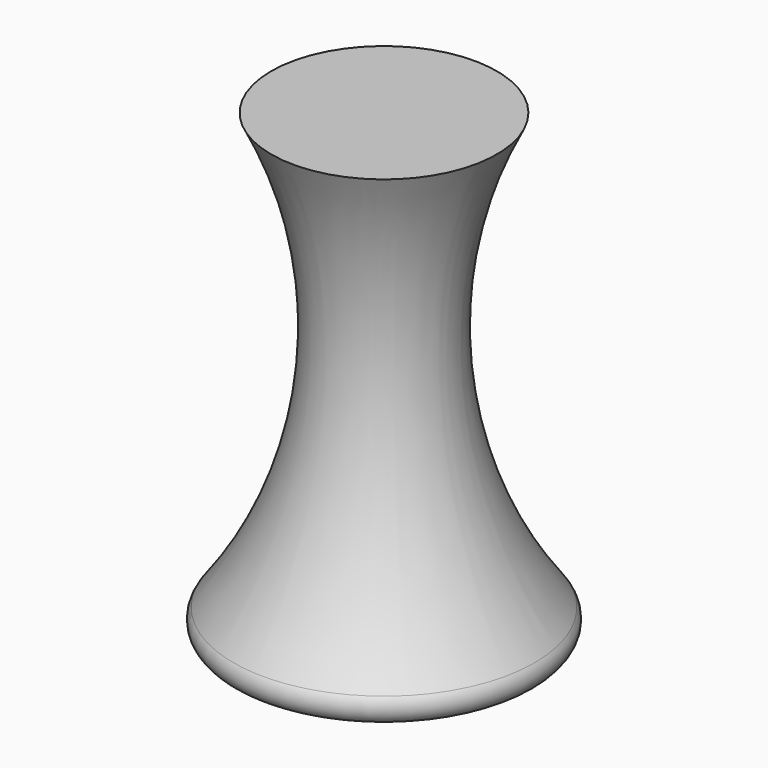
from build123d import *

# Parameters (mm, degrees)
F2_T = -7.62
F4_R = 5.08


# Not quite as in the source:
# - a fillet or chamfer that OpenCascade refuses, or shapes differently, is made with other operations: its cross-section is extruded or revolved along the edge and cut away or added


with BuildPart() as f1:
    # F0 (on Front) → F1 (revolve)
    with BuildSketch(Plane.XZ):
        with BuildLine():
            Line((143.8946140909, -50.2851232886), (143.8946140909, 51.3148767114))
            Line((143.8946140909, 51.3148767114), (119.1407005906, 51.3148767114))
            ThreePointArc((119.1407005906, 51.3148767114), (128.4046098857, -1.5785873359), (105.7946140909, -50.2851232886))
            Line((105.7946140909, -50.2851232886), (143.8946140909, -50.2851232886))
        make_face()
    revolve(axis=Axis((143.8946140909, 0, 0.5148767114), (0, 0, -1)))

    # F2
    f2_openings = [f1.faces().sort_by_distance(p)[0] for p in [
        (143.894614, 0, -50.285123),
    ]]
    offset(amount=F2_T, openings=f2_openings)

    # F3: fillet of radius 3.81 on 2 edges, made by hand

    # F3_s1 → F3_t2 (revolve, cut)
    with BuildSketch(Plane.XZ):
        with BuildLine():
            ThreePointArc((113.9178982469, -50.2855232886), (115.6120189188, -49.8884342421), (116.9532297374, -48.7798864977))
            Line((116.9532297374, -48.7798864977), (117.2567628865, -49.0105628186))
            ThreePointArc((117.2567628865, -49.0105628186), (116.6740859752, -49.7688758954), (116.0843279253, -50.5216973629))
            Line((116.0843279253, -50.5216973629), (115.7853686555, -50.6663632886))
            ThreePointArc((115.7853686555, -50.6663632886), (114.8516334512, -50.6663632886), (113.9178982469, -50.6667632886))
            Line((113.9178982469, -50.6667632886), (113.9178982469, -50.2855232886))
        make_face()
    revolve(axis=Axis((143.8946140909, 0, -50.2851232886), (0, 0, 1)), mode=Mode.SUBTRACT)

    # F3_s3 → F3_t4 (revolve, cut)
    with BuildSketch(Plane.XZ):
        with BuildLine():
            ThreePointArc((110.8854931545, -44.1691202276), (110.505670981, -48.1681963198), (113.9194373735, -50.2855232886))
            Line((113.9194373735, -50.2855232886), (113.9194373735, -50.6665904245))
            ThreePointArc((113.9194373735, -50.6665904245), (109.8570257322, -50.6661904245), (105.7946140909, -50.6661904245))
            Line((105.7946140909, -50.6661904245), (105.5128491411, -50.0285678851))
            ThreePointArc((105.5128491411, -50.0285678851), (108.1151937831, -47.039932284), (110.5820987326, -43.9385470573))
            Line((110.5820987326, -43.9385470573), (110.8854931545, -44.1691202276))
        make_face()
    revolve(axis=Axis((143.8946140909, 0, -50.2851232886), (0, 0, -1)), mode=Mode.SUBTRACT)

    # F4
    f4_edges = [f1.edges().sort_by_distance(p)[0] for p in [
        (156.981911, 0, 43.694877),
    ]]
    fillet(f4_edges, radius=F4_R)


solid = f1.part
